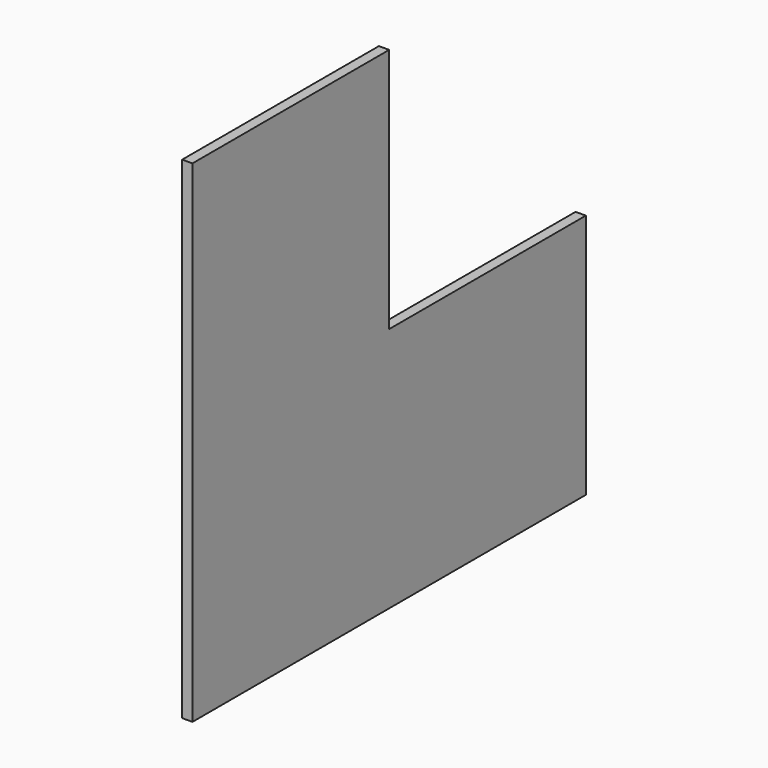
from build123d import *

# Parameters (mm, degrees)
F0_W     = 76.2
F0_H     = 76.2
F1_DEPTH = 1.5875
F2_W     = 38.1
F2_H     = 38.1
F3_DEPTH = 25.4


# Not quite as in the source:
# - a length typed as a fraction of an inch, garbled in the dataset ("3 / 203.2 mm" for 3/8 in), is restored


with BuildPart() as f1:
    # F0 (on Right) → F1 (new body)
    with BuildSketch(Plane.YZ):
        Rectangle(F0_W, F0_H)
    extrude(amount=F1_DEPTH)

    # F2 (on face) → F3 (cut)
    with BuildSketch(Plane.YZ.offset(1.5875)):
        with Locations((19.05, 19.05)):
            Rectangle(F2_W, F2_H)
    extrude(amount=-F3_DEPTH, mode=Mode.SUBTRACT)


solid = f1.part
